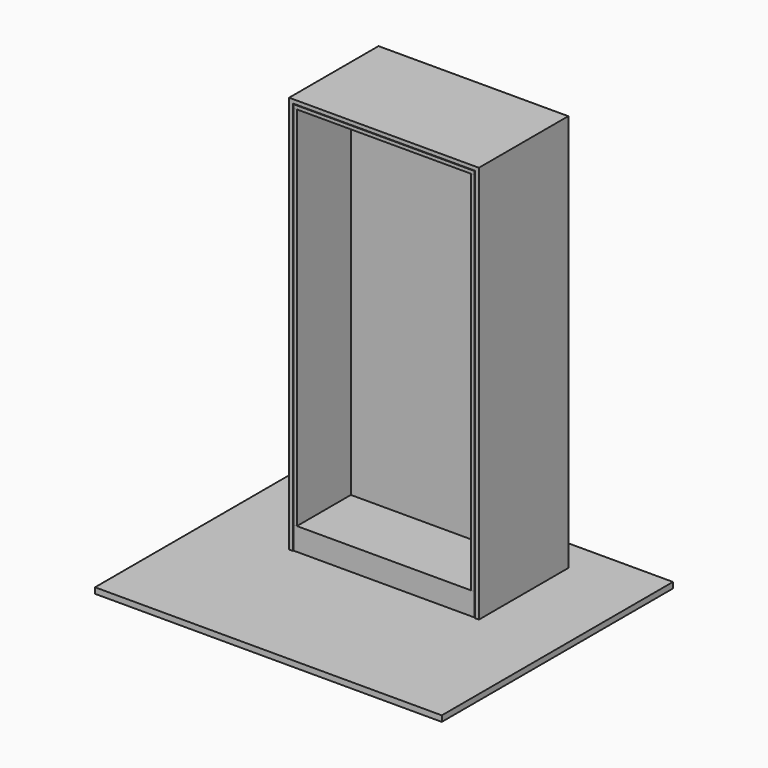
from build123d import *

# Parameters (mm, degrees)
F1_DEPTH  = 580
F3_DEPTH  = 20
F2_W      = 745
F2_H      = 1915
F2_W_2    = 805
F2_H_2    = 1975
F4_DEPTH  = 30
F5_DEPTH  = 30
F6_DEPTH  = 50
F7_W      = 1800
F7_H      = 1500
F8_DEPTH  = 30
F9_W      = 18
F9_H      = 1904
F10_DEPTH = 350
F11_DEPTH = 350
F12_START = -3
F12_DEPTH = 350
F13_DEPTH = 3
F15_DEPTH = 1904
F17_DEPTH = 18
F19_DEPTH = 18
F20_W     = 871.785590257
F20_H     = 3
F21_DEPTH = 1922


with BuildPart() as f1:
    # F0 (on Front) → F1 (new body)
    with BuildSketch(Plane.XZ):
        Polygon((-492.5, -1022.5), (-472.5, -1022.5), (-472.5, 1022.5), (472.5, 1022.5), (472.5, -1022.5), (492.5, -1022.5), (492.5, 1042.5), (-492.5, 1042.5), align=None)
    extrude(amount=F1_DEPTH)

    # F2 (on Front) → F3 (join)
    with BuildSketch(Plane.XZ):
        Polygon((-402.5, -1022.5), (-402.5, 952.5), (402.5, 952.5), (402.5, -1022.5), (472.5, -1022.5), (472.5, 1022.5), (-472.5, 1022.5), (-472.5, -1022.5), align=None)
    extrude(amount=F3_DEPTH)

    # F2 (on Front) → F4 (join)
    with BuildSketch(Plane.XZ):
        with Locations((0, -35)):
            Rectangle(F2_W_2, F2_H_2)
        with Locations((0, -35)):
            Rectangle(F2_W, F2_H, mode=Mode.SUBTRACT)
    extrude(amount=F4_DEPTH)

    # F7 (on face) → F8 (join)
    with BuildSketch(Plane(origin=(0, 0, -1022.5), x_dir=(1, 0, 0), z_dir=(0, 0, -1))):
        with Locations((0, 580)):
            Rectangle(F7_W, F7_H)
    extrude(amount=F8_DEPTH)


with BuildPart() as f3:
    # F2 (on Front) → F3, piece 2 (new body)
    with BuildSketch(Plane.XZ):
        with Locations((0, -35)):
            Rectangle(F2_W, F2_H)
        with BuildLine():
            ThreePointArc((322.5, 25), (340.1776695297, 17.6776695297), (347.5, 0))
            ThreePointArc((347.5, 0), (322.5, -25), (297.5, 0))
            Line((297.5, 0), (232.5, 0))
            ThreePointArc((232.5, 0), (225.4289321881, 2.9289321881), (222.5, 10))
            Line((222.5, 10), (222.5, 15))
            ThreePointArc((222.5, 15), (225.4289321881, 22.0710678119), (232.5, 25))
            Line((232.5, 25), (322.5, 25))
        make_face(mode=Mode.SUBTRACT)
    extrude(amount=F3_DEPTH)

    # F2 (on Front) → F5 (join)
    with BuildSketch(Plane.XZ):
        with BuildLine():
            ThreePointArc((297.5, 0), (322.5, -25), (347.5, 0))
            ThreePointArc((347.5, 0), (340.1776695297, 17.6776695297), (322.5, 25))
            Line((322.5, 25), (322.5, 0))
            Line((322.5, 0), (297.5, 0))
        make_face()
    extrude(amount=F5_DEPTH)

    # F2 (on Front) → F6 (join)
    with BuildSketch(Plane.XZ):
        with BuildLine():
            ThreePointArc((297.5, 0), (304.8223304703, 17.6776695297), (322.5, 25))
            Line((322.5, 25), (232.5, 25))
            ThreePointArc((232.5, 25), (225.4289321881, 22.0710678119), (222.5, 15))
            Line((222.5, 15), (222.5, 10))
            ThreePointArc((222.5, 10), (225.4289321881, 2.9289321881), (232.5, 0))
            Line((232.5, 0), (297.5, 0))
        make_face()
        with BuildLine():
            Line((322.5, 0), (322.5, 25))
            ThreePointArc((322.5, 25), (304.8223304703, 17.6776695297), (297.5, 0))
            Line((297.5, 0), (322.5, 0))
        make_face()
    extrude(amount=F6_DEPTH)


with BuildPart() as f10:
    # F9 (on face) → F10 (new body)
    with BuildSketch(Plane.XZ.offset(580)):
        with Locations((-461, 50)):
            Rectangle(F9_W, F9_H)
    extrude(amount=-F10_DEPTH)


with BuildPart() as f11:
    # F9 (on face) → F11 (new body)
    with BuildSketch(Plane.XZ.offset(580)):
        Polygon((470, 1002), (470, 1020), (-470, 1020), (-470, 1002), (-452, 1002), (452, 1002), align=None)
    extrude(amount=-F11_DEPTH)

    # F18 (on face) → F19 (cut, through all)
    with BuildSketch(Plane(origin=(0, 0, 1002), x_dir=(1, 0, 0), z_dir=(0, 0, -1))):
        Polygon((470, 230), (470, 580), (401.785590257, 230), align=None)
    extrude(amount=-F19_DEPTH, mode=Mode.SUBTRACT)


with BuildPart() as f12:
    # F9 (on face) → F12 (new body)
    with BuildSketch(Plane.XZ.offset(580).offset(F12_START)):
        Polygon((470, -920), (470, -902), (452, -902), (-452, -902), (-470, -902), (-470, -920), (-452, -920), (452, -920), align=None)
    extrude(amount=-F12_DEPTH)

    # F16 (on face) → F17 (cut, through all)
    with BuildSketch(Plane.XY.offset(-902)):
        Polygon((470, -580), (470, -227), (401.2008953163, -227), align=None)
    extrude(amount=-F17_DEPTH, mode=Mode.SUBTRACT)


with BuildPart() as f13:
    # F9 (on face) → F13 (new body)
    with BuildSketch(Plane.XZ.offset(580)):
        Polygon((470, -920), (470, -902), (452, -902), (-452, -902), (-470, -902), (-470, -920), (-452, -920), (452, -920), align=None)
        Polygon((470, -1020), (470, -920), (452, -920), (-452, -920), (-470, -920), (-470, -1020), align=None)
    extrude(amount=-F13_DEPTH)


with BuildPart() as f15:
    # F14 (on face) → F15 (new body, through all)
    with BuildSketch(Plane.XY.offset(-902)):
        Polygon((452, -580), (470, -580), (469.4153050593, -577), (451.4153050593, -577), align=None)
        Polygon((469.4153050593, -577), (401.785590257, -230), (383.785590257, -230), (451.4153050593, -577), align=None)
    extrude(amount=F15_DEPTH)


with BuildPart() as f21:
    # F20 (on face) → F21 (new body, through all)
    with BuildSketch(Plane.XY.offset(-902)):
        with Locations((-34.1072048715, -228.5)):
            Rectangle(F20_W, F20_H)
    extrude(amount=F21_DEPTH)


solid = Compound([f1.part, f3.part, f10.part, f11.part, f12.part, f13.part, f15.part, f21.part])
